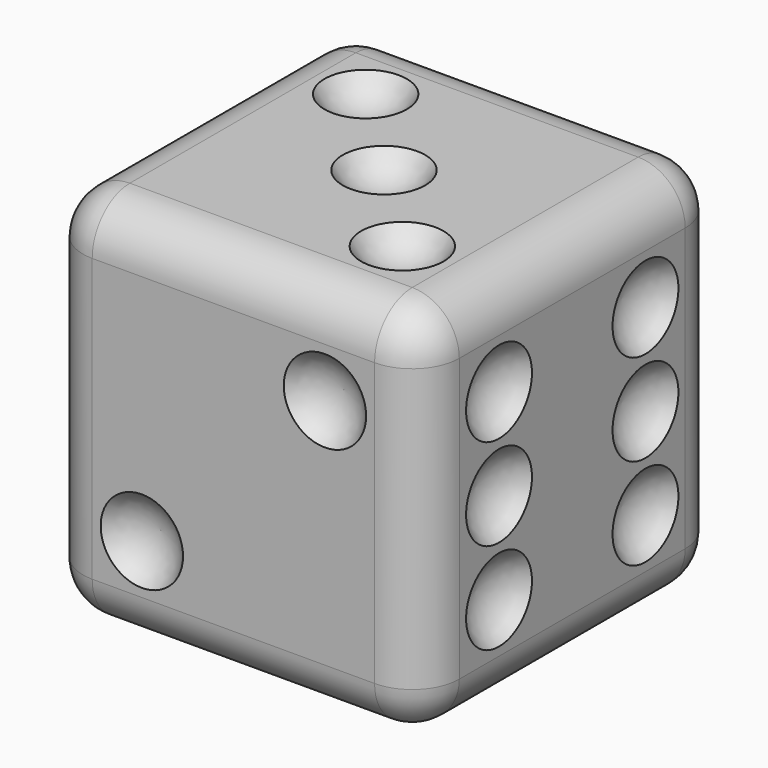
from build123d import *

# Parameters (mm, degrees)
F0_W      = 16
F0_H      = 16
F1_DEPTH  = 16
F2_R      = 2
F3_R      = 1.75
F4_DEPTH  = 1
F8_R      = 1.75
F8_R_2    = 1.7502183246
F9_DEPTH  = 1
F11_R     = 1.75
F12_DEPTH = 1
F14_R     = 1.75
F15_DEPTH = 1
F17_R     = 1.75
F18_DEPTH = 1
F20_R     = 1.75
F21_DEPTH = 1


# Not quite as in the source:
# - a fillet or chamfer that OpenCascade refuses, or shapes differently, is made with other operations: its cross-section is extruded or revolved along the edge and cut away or added


with BuildPart() as f1:
    # F0 (on Top) → F1 (new body)
    with BuildSketch(Plane.XY):
        Rectangle(F0_W, F0_H)
    extrude(amount=-F1_DEPTH)

    # F2
    f2_edges = [f1.edges().sort_by_distance(p)[0] for p in [
        (0, -8, 0),
        (-8, 0, 0),
        (0, 8, 0),
        (8, 0, 0),
        (8, -8, -8),
        (8, 8, -8),
        (8, 0, -16),
        (0, 8, -16),
        (-8, 8, -8),
        (-8, 0, -16),
        (-8, -8, -8),
        (0, -8, -16),
    ]]
    fillet(f2_edges, radius=F2_R)

    # F3 (on face) → F4 (cut)
    with BuildSketch(Plane.XY):
        Circle(F3_R)
        with Locations((3.89, -3.8881743788)):
            Circle(F3_R)
        with Locations((-3.89, 3.8881743788)):
            Circle(F3_R)
    extrude(amount=-F4_DEPTH, mode=Mode.SUBTRACT)

    # F5: fillet of radius 2.016187672 on 1 edges, made by hand

    # F5_s1 → F5_t2 (revolve)
    with BuildSketch(Plane.XZ.offset(3.8881743788)):
        with BuildLine():
            ThreePointArc((5.64, 0), (4.9026670776, -0.7322169988), (3.8986283154, -1))
            Line((3.8986283154, -1), (5.64, -1))
            Line((5.64, -1), (5.64, 0))
        make_face()
    revolve(axis=Axis((3.89, -3.8881743788, -1), (0, 0, 1)))

    # F6: fillet of radius 2.016187672 on 1 edges, made by hand

    # F6_s1 → F6_t2 (revolve)
    with BuildSketch(Plane.XZ):
        with BuildLine():
            ThreePointArc((1.75, 0), (1.0126670776, -0.7322169988), (0.0086283154, -1))
            Line((0.0086283154, -1), (1.75, -1))
            Line((1.75, -1), (1.75, 0))
        make_face()
    revolve(axis=Axis((0, 0, -1), (0, 0, 1)))

    # F7: fillet of radius 2.016187672 on 1 edges, made by hand

    # F7_s1 → F7_t2 (revolve)
    with BuildSketch(Plane.XZ.offset(-3.8881743788)):
        with BuildLine():
            ThreePointArc((-2.14, 0), (-2.8773329224, -0.7322169988), (-3.8813716846, -1))
            Line((-3.8813716846, -1), (-2.14, -1))
            Line((-2.14, -1), (-2.14, 0))
        make_face()
    revolve(axis=Axis((-3.89, 3.8881743788, -1), (0, 0, 1)))

    # F8 (on face) → F9 (cut)
    with BuildSketch(Plane(origin=(0, 0, -16), x_dir=(1, 0, 0), z_dir=(0, 0, -1))):
        with Locations((-3.8887145573, 3.88946)):
            Circle(F8_R)
        with Locations((3.88946, 3.8887145573)):
            Circle(F8_R)
        with Locations((-3.8892416754, -3.8892416754)):
            Circle(F8_R_2)
        with Locations((3.8892416754, -3.8892416754)):
            Circle(F8_R_2)
    extrude(amount=-F9_DEPTH, mode=Mode.SUBTRACT)

    # F10: fillet of radius 2.016187672 on 4 edges, made by hand

    # F10_s1 → F10_t2 (revolve)
    with BuildSketch(Plane.XZ.offset(3.88946)):
        with BuildLine():
            ThreePointArc((-2.1387145573, -16), (-2.8760474797, -15.2677830012), (-3.8800862419, -15))
            Line((-3.8800862419, -15), (-2.1387145573, -15))
            Line((-2.1387145573, -15), (-2.1387145573, -16))
        make_face()
    revolve(axis=Axis((-3.8887145573, -3.88946, -15), (0, 0, -1)))

    # F10_s3 → F10_t4 (revolve)
    with BuildSketch(Plane.XZ.offset(3.8887145573)):
        with BuildLine():
            ThreePointArc((5.63946, -16), (4.9021270776, -15.2677830012), (3.8980883154, -15))
            Line((3.8980883154, -15), (5.63946, -15))
            Line((5.63946, -15), (5.63946, -16))
        make_face()
    revolve(axis=Axis((3.88946, -3.8887145573, -15), (0, 0, -1)))

    # F10_s5 → F10_t6 (revolve)
    with BuildSketch(Plane.XZ.offset(-3.8892416754)):
        with BuildLine():
            ThreePointArc((-2.1390233507, -16), (-2.8763562731, -15.2677830012), (-3.8803950353, -15))
            Line((-3.8803950353, -15), (-2.1390233507, -15))
            Line((-2.1390233507, -15), (-2.1390233507, -16))
        make_face()
    revolve(axis=Axis((-3.8892416754, 3.8892416754, -15), (0, 0, -1)))

    # F10_s7 → F10_t8 (revolve)
    with BuildSketch(Plane.XZ.offset(-3.8892416754)):
        with BuildLine():
            ThreePointArc((5.63946, -16), (4.9021270776, -15.2677830012), (3.8980883154, -15))
            Line((3.8980883154, -15), (5.63946, -15))
            Line((5.63946, -15), (5.63946, -16))
        make_face()
    revolve(axis=Axis((3.8892416754, 3.8892416754, -15), (0, 0, -1)))

    # F11 (on face) → F12 (cut)
    with BuildSketch(Plane(origin=(0, 8, 0), x_dir=(-1, 0, 0), z_dir=(0, 1, 0))):
        with Locations((0, -8)):
            Circle(F11_R)
        with Locations((-3.88946, -4.11)):
            Circle(F11_R)
        with Locations((-3.88946, -11.88946)):
            Circle(F11_R)
        with Locations((3.88946, -11.88946)):
            Circle(F11_R)
        with Locations((3.88946, -4.11054)):
            Circle(F11_R)
    extrude(amount=-F12_DEPTH, mode=Mode.SUBTRACT)

    # F13: fillet of radius 2.016187672 on 5 edges, made by hand

    # F13_s1 → F13_t2 (revolve)
    with BuildSketch(Plane.XY.offset(-4.11)):
        with BuildLine():
            ThreePointArc((2.13946, 8), (2.8767929224, 7.2677830012), (3.8808316846, 7))
            Line((3.8808316846, 7), (2.13946, 7))
            Line((2.13946, 7), (2.13946, 8))
        make_face()
    revolve(axis=Axis((3.88946, 7, -4.11), (0, 1, 0)))

    # F13_s3 → F13_t4 (revolve)
    with BuildSketch(Plane.XY.offset(-8)):
        with BuildLine():
            ThreePointArc((-1.75, 8), (-1.0126670776, 7.2677830012), (-0.0086283154, 7))
            Line((-0.0086283154, 7), (-1.75, 7))
            Line((-1.75, 7), (-1.75, 8))
        make_face()
    revolve(axis=Axis((0, 7, -8), (0, 1, 0)))

    # F13_s5 → F13_t6 (revolve)
    with BuildSketch(Plane.XY.offset(-11.88946)):
        with BuildLine():
            ThreePointArc((2.13946, 8), (2.8767929224, 7.2677830012), (3.8808316846, 7))
            Line((3.8808316846, 7), (2.13946, 7))
            Line((2.13946, 7), (2.13946, 8))
        make_face()
    revolve(axis=Axis((3.88946, 7, -11.88946), (0, 1, 0)))

    # F13_s7 → F13_t8 (revolve)
    with BuildSketch(Plane.XY.offset(-11.88946)):
        with BuildLine():
            ThreePointArc((-5.63946, 8), (-4.9021270776, 7.2677830012), (-3.8980883154, 7))
            Line((-3.8980883154, 7), (-5.63946, 7))
            Line((-5.63946, 7), (-5.63946, 8))
        make_face()
    revolve(axis=Axis((-3.88946, 7, -11.88946), (0, 1, 0)))

    # F13_s9 → F13_t10 (revolve)
    with BuildSketch(Plane.XY.offset(-4.11054)):
        with BuildLine():
            ThreePointArc((-5.63946, 8), (-4.9021270776, 7.2677830012), (-3.8980883154, 7))
            Line((-3.8980883154, 7), (-5.63946, 7))
            Line((-5.63946, 7), (-5.63946, 8))
        make_face()
    revolve(axis=Axis((-3.88946, 7, -4.11054), (0, 1, 0)))

    # F14 (on face) → F15 (cut)
    with BuildSketch(Plane.YZ.offset(8)):
        with Locations((3.89, -4.11)):
            Circle(F14_R)
        with Locations((3.89, -8)):
            Circle(F14_R)
        with Locations((3.89, -11.89)):
            Circle(F14_R)
        with Locations((-3.89, -8)):
            Circle(F14_R)
        with Locations((-3.89, -4.11)):
            Circle(F14_R)
        with Locations((-3.89, -11.89)):
            Circle(F14_R)
    extrude(amount=-F15_DEPTH, mode=Mode.SUBTRACT)

    # F16: fillet of radius 2.016187672 on 6 edges, made by hand

    # F16_s1 → F16_t2 (revolve)
    with BuildSketch(Plane.XY.offset(-11.89)):
        with BuildLine():
            ThreePointArc((8, -2.14), (7.2677830012, -2.8773329224), (7, -3.8813716846))
            Line((7, -3.8813716846), (7, -2.14))
            Line((7, -2.14), (8, -2.14))
        make_face()
    revolve(axis=Axis((7, -3.89, -11.89), (1, 0, 0)))

    # F16_s3 → F16_t4 (revolve)
    with BuildSketch(Plane.XY.offset(-8)):
        with BuildLine():
            ThreePointArc((8, -2.14), (7.2677830012, -2.8773329224), (7, -3.8813716846))
            Line((7, -3.8813716846), (7, -2.14))
            Line((7, -2.14), (8, -2.14))
        make_face()
    revolve(axis=Axis((7, -3.89, -8), (1, 0, 0)))

    # F16_s5 → F16_t6 (revolve)
    with BuildSketch(Plane.XY.offset(-4.11)):
        with BuildLine():
            ThreePointArc((8, -2.14), (7.2677830012, -2.8773329224), (7, -3.8813716846))
            Line((7, -3.8813716846), (7, -2.14))
            Line((7, -2.14), (8, -2.14))
        make_face()
    revolve(axis=Axis((7, -3.89, -4.11), (1, 0, 0)))

    # F16_s7 → F16_t8 (revolve)
    with BuildSketch(Plane.XY.offset(-8)):
        with BuildLine():
            ThreePointArc((8, 5.64), (7.2677830012, 4.9026670776), (7, 3.8986283154))
            Line((7, 3.8986283154), (7, 5.64))
            Line((7, 5.64), (8, 5.64))
        make_face()
    revolve(axis=Axis((7, 3.89, -8), (1, 0, 0)))

    # F16_s9 → F16_t10 (revolve)
    with BuildSketch(Plane.XY.offset(-11.89)):
        with BuildLine():
            ThreePointArc((8, 5.64), (7.2677830012, 4.9026670776), (7, 3.8986283154))
            Line((7, 3.8986283154), (7, 5.64))
            Line((7, 5.64), (8, 5.64))
        make_face()
    revolve(axis=Axis((7, 3.89, -11.89), (1, 0, 0)))

    # F16_s11 → F16_t12 (revolve)
    with BuildSketch(Plane.XY.offset(-4.11)):
        with BuildLine():
            ThreePointArc((8, 5.64), (7.2677830012, 4.9026670776), (7, 3.8986283154))
            Line((7, 3.8986283154), (7, 5.64))
            Line((7, 5.64), (8, 5.64))
        make_face()
    revolve(axis=Axis((7, 3.89, -4.11), (1, 0, 0)))

    # F17 (on face) → F18 (cut)
    with BuildSketch(Plane(origin=(-8, 0, 0), x_dir=(0, -1, 0), z_dir=(-1, 0, 0))):
        with Locations((0, -8)):
            Circle(F17_R)
    extrude(amount=-F18_DEPTH, mode=Mode.SUBTRACT)

    # F19: fillet of radius 2.016187672 on 1 edges, made by hand

    # F19_s1 → F19_t2 (revolve)
    with BuildSketch(Plane.XY.offset(-8)):
        with BuildLine():
            ThreePointArc((-8, -1.75), (-7.2677830012, -1.0126670776), (-7, -0.0086283154))
            Line((-7, -0.0086283154), (-7, -1.75))
            Line((-7, -1.75), (-8, -1.75))
        make_face()
    revolve(axis=Axis((-7, 0, -8), (-1, 0, 0)))

    # F20 (on face) → F21 (cut)
    with BuildSketch(Plane.XZ.offset(8)):
        with Locations((-3.89, -11.89)):
            Circle(F20_R)
        with Locations((3.89, -4.11)):
            Circle(F20_R)
    extrude(amount=-F21_DEPTH, mode=Mode.SUBTRACT)

    # F22: fillet of radius 2.016187672 on 2 edges, made by hand

    # F22_s1 → F22_t2 (revolve)
    with BuildSketch(Plane.XY.offset(-11.89)):
        with BuildLine():
            ThreePointArc((-2.14, -8), (-2.8773329224, -7.2677830012), (-3.8813716846, -7))
            Line((-3.8813716846, -7), (-2.14, -7))
            Line((-2.14, -7), (-2.14, -8))
        make_face()
    revolve(axis=Axis((-3.89, -7, -11.89), (0, -1, 0)))

    # F22_s3 → F22_t4 (revolve)
    with BuildSketch(Plane.XY.offset(-4.11)):
        with BuildLine():
            ThreePointArc((5.64, -8), (4.9026670776, -7.2677830012), (3.8986283154, -7))
            Line((3.8986283154, -7), (5.64, -7))
            Line((5.64, -7), (5.64, -8))
        make_face()
    revolve(axis=Axis((3.89, -7, -4.11), (0, -1, 0)))


solid = f1.part
